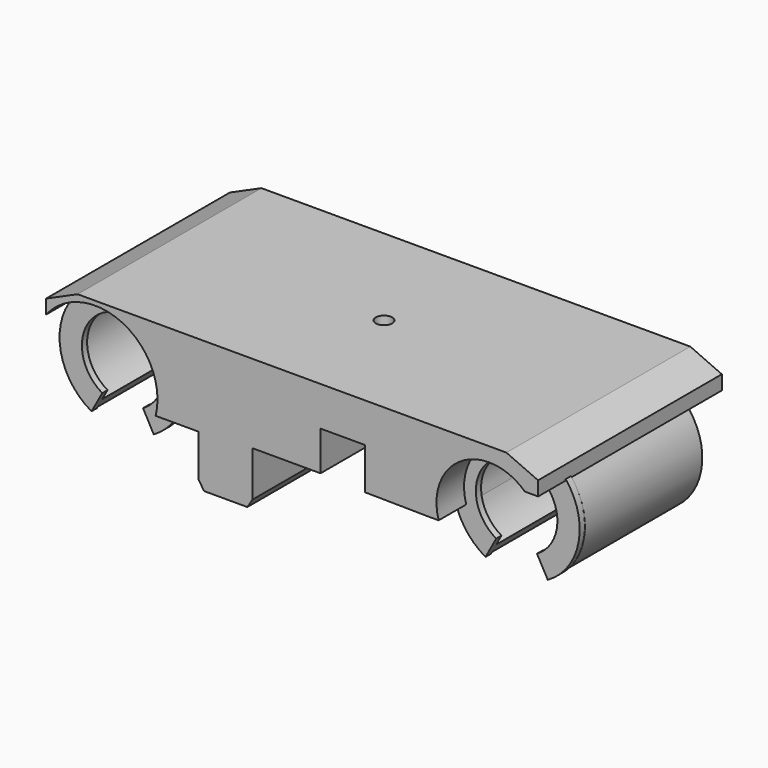
from build123d import *

# Parameters (mm, degrees)
F1_DEPTH = 35
F2_DEPTH = 22.5
F5_DEPTH = 2
F7_D     = 2.4
F7_DEPTH = 18
F7_TIP   = 0.7210327428
F10_D    = 5


with BuildPart() as f1:
    # F0 (on Front) → F1 (new body, symmetric)
    with BuildSketch(Plane.XZ):
        with BuildLine():
            ThreePointArc((-74.9516211859, 11.7238655704), (-51.6668855763, 17.075104802), (-41.558504512, -4.5728813857))
            Line((-41.558504512, -4.5728813857), (-28.4346174449, -4.5728813857))
            Line((-28.4346174449, -4.5728813857), (-28.4346174449, -17.4488071352))
            Line((-28.4346174449, -17.4488071352), (-26.8566174449, -19.9622381479))
            Line((-26.8566174449, -19.9622381479), (-13.633294031, -19.9622381479))
            Line((-13.633294031, -19.9622381479), (-12.0557677819, -17.4488071352))
            Line((-12.0557677819, -17.4488071352), (-12.0557677819, -3.6602381479))
            Line((-12.0557677819, -3.6602381479), (8.6728588212, -3.6602381479))
            Line((8.6728588212, -3.6602381479), (8.6728588212, 8.3482577465))
            Line((8.6728588212, 8.3482577465), (22.1839677542, 8.3482577465))
            Line((22.1839677542, 8.3482577465), (22.1839677542, -4.337257977))
            Line((22.1839677542, -4.337257977), (41.558504512, -4.5728813857))
            Line((41.558504512, -4.5728813857), (44.6673956605, -4.5728813857))
            ThreePointArc((44.6673956605, -4.5728813857), (51.5748749774, 13.6021052912), (70.9240066517, 11.6904267961))
            Line((70.9240066517, 11.6904267961), (74.9777809213, 11.6904267961))
            Line((74.9777809213, 11.6904267961), (74.9516211859, 16.0203691918))
            Line((74.9516211859, 16.0203691918), (65.3270802818, 20.3168728132))
            Line((65.3270802818, 20.3168728132), (-65.3270802818, 20.3168728132))
            Line((-65.3270802818, 20.3168728132), (-74.9516211859, 16.0203691918))
            Line((-74.9516211859, 16.0203691918), (-74.9516211859, 11.7238655704))
        make_face()
    extrude(amount=F1_DEPTH, both=True)

    # F0 (on Front) → F2 (join, symmetric)
    with BuildSketch(Plane.XZ):
        with BuildLine():
            ThreePointArc((-68, -13.8564064606), (-75.8989864476, -1.7950570853), (-70.888111686, 11.7238655704))
            Line((-70.888111686, 11.7238655704), (-74.9516211859, 11.7238655704))
            ThreePointArc((-74.9516211859, 11.7238655704), (-78.6540953163, -3.6089787931), (-69.5, -16.4544826719))
            Line((-69.5, -16.4544826719), (-68, -13.8564064606))
        make_face()
        with BuildLine():
            ThreePointArc((-44.6673956605, -4.5728813857), (-47.4441819952, -9.9172291609), (-52, -13.8564064606))
            Line((-52, -13.8564064606), (-50.5, -16.4544826719))
            ThreePointArc((-50.5, -16.4544826719), (-44.818600038, -11.4247579927), (-41.558504512, -4.5728813857))
            Line((-41.558504512, -4.5728813857), (-44.6673956605, -4.5728813857))
        make_face()
        with BuildLine():
            ThreePointArc((-70.888111686, 11.7238655704), (-51.5540323778, 13.5891732981), (-44.6673956605, -4.5728813857))
            Line((-44.6673956605, -4.5728813857), (-41.558504512, -4.5728813857))
            ThreePointArc((-41.558504512, -4.5728813857), (-51.6668855763, 17.075104802), (-74.9516211859, 11.7238655704))
            Line((-74.9516211859, 11.7238655704), (-70.888111686, 11.7238655704))
        make_face()
        with BuildLine():
            ThreePointArc((52, -13.8564064606), (47.4441819952, -9.9172291609), (44.6673956605, -4.5728813857))
            Line((44.6673956605, -4.5728813857), (41.558504512, -4.5728813857))
            ThreePointArc((41.558504512, -4.5728813857), (44.818600038, -11.4247579927), (50.5, -16.4544826719))
            Line((50.5, -16.4544826719), (52, -13.8564064606))
        make_face()
        with BuildLine():
            ThreePointArc((69.5, -16.4544826719), (78.6500515267, -3.629817909), (74.9777809213, 11.6904267961))
            Line((74.9777809213, 11.6904267961), (70.9240066517, 11.6904267961))
            ThreePointArc((70.9240066517, 11.6904267961), (75.8962158798, -1.8194286745), (68, -13.8564064606))
            Line((68, -13.8564064606), (69.5, -16.4544826719))
        make_face()
    extrude(amount=F2_DEPTH, both=True)

    # F4 (on offset) → F5 (join)
    with BuildSketch(Plane.XZ.offset(22.5)):
        with BuildLine():
            ThreePointArc((-66.2250077663, -10.764406164), (-60.0242756476, 12.4257611455), (-53.8000638867, -10.7581152906))
            Line((-53.8000638867, -10.7581152906), (-50.5566579219, -16.7363728506))
            ThreePointArc((-50.5566579219, -16.7363728506), (-59.9985634557, 19.2255688342), (-69.5131042914, -16.7172238027))
            Line((-69.5131042914, -16.7172238027), (-66.2250077663, -10.764406164))
        make_face()
        with BuildLine():
            ThreePointArc((69.5131042914, -16.7172238027), (59.9985634557, 19.2255688342), (50.5566579219, -16.7363728506))
            Line((50.5566579219, -16.7363728506), (53.8000638867, -10.7581152906))
            ThreePointArc((53.8000638867, -10.7581152906), (60.0242756476, 12.4257611455), (66.2250077663, -10.764406164))
            Line((66.2250077663, -10.764406164), (69.5131042914, -16.7172238027))
        make_face()
    extrude(amount=F5_DEPTH)

    # F7 (one way)
    with BuildSketch(Plane.YZ.offset(-12.0557677819)):
        with Locations((-20, -11.9100315496), (20, -11.9100315496)):
            Circle(F7_D / 2)
    extrude(amount=-F7_DEPTH, mode=Mode.SUBTRACT)
    with Locations(Plane.YZ.offset(-12.0557677819)):
        with Locations((-20, -11.9100315496), (20, -11.9100315496)):
            with Locations((0, 0, -(F7_DEPTH + F7_TIP / 2))):  # 118° drill point
                Cone(0, F7_D / 2, F7_TIP, mode=Mode.SUBTRACT)

    # F10 (through all)
    with Locations(Plane.XY.offset(20.3168728132)):
        with Locations((0, 0)):
            Hole(F10_D / 2)


solid = f1.part
